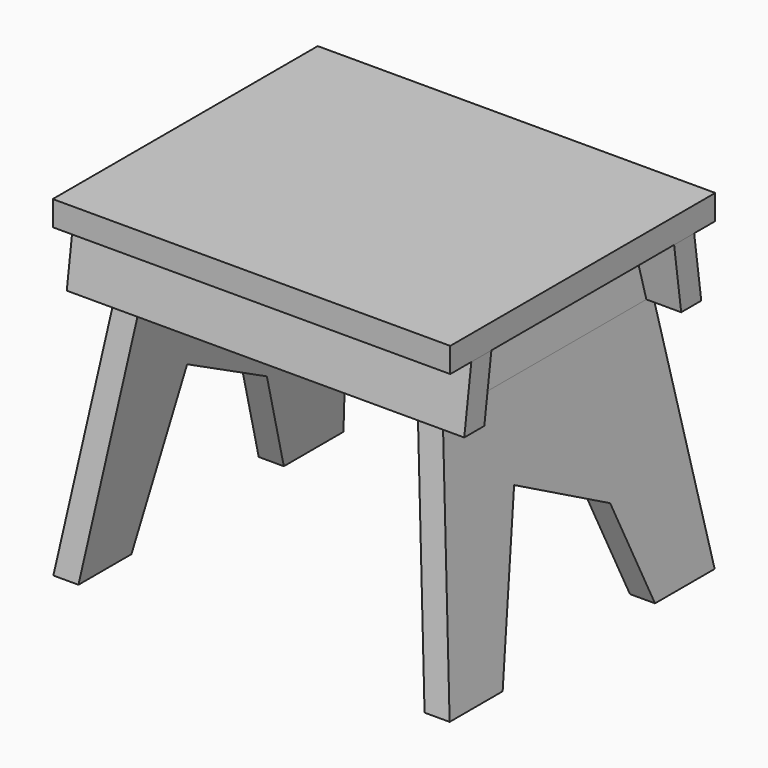
from build123d import *

# Parameters (mm, degrees)
F1_DEPTH      = 127
F2_DEPTH      = 127
F2_DEPTH_BACK = 127
F4_DEPTH      = 152.401
F4_DEPTH_BACK = 152.401
F6_DEPTH      = 152.4
F6_DEPTH_BACK = 152.4


# Not quite as in the source:
# - a feature names something its author has since deleted; it is built from what else it names


with BuildPart() as f1:
    # F0 (on Front) → F1 (new body, symmetric)
    with BuildSketch(Plane.XZ):
        Polygon((152.4, -9.525), (152.4, 9.525), (-152.4, 9.525), (-152.4, -9.525), (-151.9371964019, -9.525), (-141.1124509845, -9.525), (-118.9171865446, -9.525), (-99.6799712881, -9.525), (99.6799712881, -9.525), (118.9171865446, -9.525), (141.1124509845, -9.525), (151.9371964019, -9.525), align=None)
    extrude(amount=F1_DEPTH, both=True)


with BuildPart() as f2:
    # F0 (on Front) → F2 (new body, two sides)
    with BuildSketch(Plane.XZ) as f2_sk:
        Polygon((-99.6799712881, -9.525), (-118.9171865446, -9.525), (-125.6996872273, -57.785), (-106.4624719709, -57.785), align=None)
        Polygon((-106.4624719709, -57.785), (-125.6996872273, -57.785), (-151.9371964019, -244.4745783714), (-132.6999811454, -244.4745783714), align=None)
    extrude(amount=F2_DEPTH)
    extrude(f2_sk.sketch, amount=-F2_DEPTH_BACK)


with BuildPart() as f2b:
    # F0 (on Front) → F2, piece 2 (new body, two sides)
    with BuildSketch(Plane.XZ) as f2_2_sk:
        Polygon((125.6996872273, -57.785), (118.9171865446, -9.525), (99.6799712881, -9.525), (106.4624719709, -57.785), align=None)
        Polygon((151.9371964019, -244.4745783714), (125.6996872273, -57.785), (106.4624719709, -57.785), (132.6999811454, -244.4745783714), align=None)
    extrude(amount=F2_DEPTH)
    extrude(f2_2_sk.sketch, amount=-F2_DEPTH_BACK)


with BuildPart() as f4_tool:
    # F3 (on Right) → F4 (new body, two sides)
    with BuildSketch(Plane.YZ) as f4_sk:
        Polygon((-76.2000000004, -244.4745783714), (69.8500000004, -244.4745783714), (40.2337837021, -168.2745783714), (-44.0084859729, -123.8245783714), align=None)
        Polygon((126.9999999998, -244.4745783714), (126.9999999997, -9.525), (93.9799901431, -9.525), align=None)
        Polygon((-127.0000000004, -244.4745783714), (-93.9799901431, -9.525), (-127.0000000004, -9.525), align=None)
    extrude(amount=-F4_DEPTH)
    extrude(f4_sk.sketch, amount=F4_DEPTH_BACK)


with BuildPart() as f2_1:
    add(f2.part)

    # F4: cut by f4_tool
    add(f4_tool.part, mode=Mode.SUBTRACT)


with BuildPart() as f2b_1:
    add(f2b.part)

    # F4: cut by f4_tool
    add(f4_tool.part, mode=Mode.SUBTRACT)


with BuildPart() as f6:
    # F5 (on Right) → F6 (new body, two sides)
    with BuildSketch(Plane.YZ) as f6_sk:
        Polygon((-93.9799901431, -9.525), (-106.8048003141, -9.525), (-113.5873009968, -57.785), (-100.7624908258, -57.785), align=None)
        Polygon((-87.5675850576, -9.525), (-93.9799901431, -9.525), (-100.7624908258, -57.785), (-94.3500857403, -57.785), align=None)
    extrude(amount=F6_DEPTH)
    extrude(f6_sk.sketch, amount=-F6_DEPTH_BACK)


with BuildPart() as f6b:
    # F5 (on Right) → F6, piece 2 (new body, two sides)
    with BuildSketch(Plane.YZ) as f6_2_sk:
        Polygon((106.8048003141, -9.525), (93.9799901431, -9.525), (100.7624908258, -57.785), (113.5873009968, -57.785), align=None)
        Polygon((93.9799901431, -9.525), (87.5675850576, -9.525), (94.3500857403, -57.785), (100.7624908258, -57.785), align=None)
    extrude(amount=F6_DEPTH)
    extrude(f6_2_sk.sketch, amount=-F6_DEPTH_BACK)


solid = Compound([f1.part, f2_1.part, f2b_1.part, f6.part, f6b.part])
